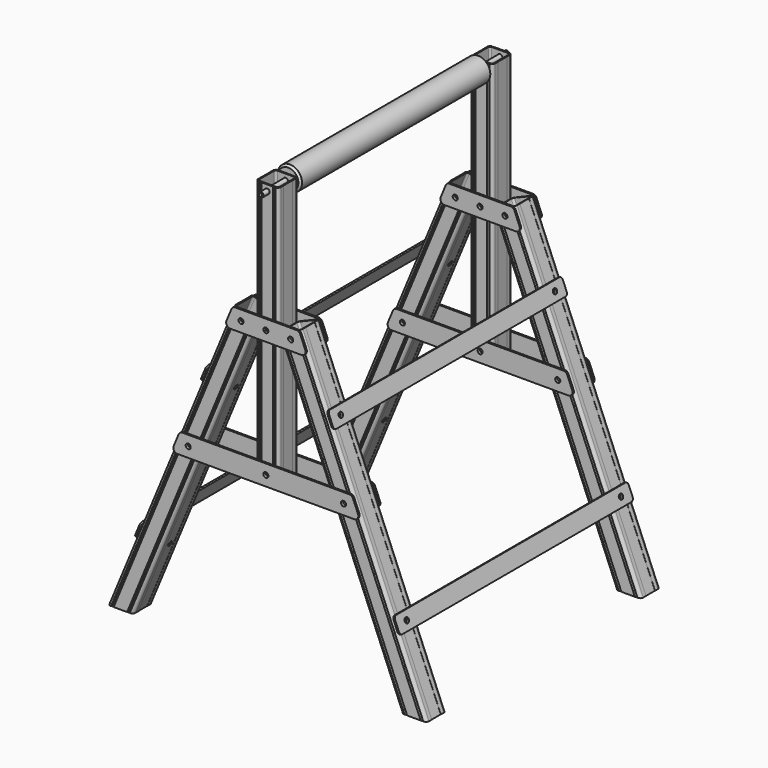
from build123d import *

# Parameters (mm, degrees)
F0_R      = 6.25
F1_DEPTH  = 60
F2_R      = 7.5
F4_REACH  = 887.042655099
F5_R      = 6.25
F6_DEPTH  = 57.7
F7_W      = 55.7
F7_H      = 653.8274706661
F7_R      = 6.25
F8_DEPTH  = 60
F9_R      = 7.5
F11_DEPTH = 653.8274706661
F14_R     = 6.25
F15_DEPTH = 4
F16_R     = 10
F16_2_R   = 10
F21_R     = 5.9
F22_DEPTH = 380
F23_R     = 30
F23_R_2   = 6.25
F24_DEPTH = 295
F25_SIZE  = 2
F26_SIZE  = 5
F28_W     = 720
F28_H     = 40
F28_R     = 6.25
F29_DEPTH = 4
F30_R     = 7.5
F30_2_R   = 7.5


# Not quite as in the source:
# - a feature names something its author has since deleted; it is built from what else it names


with BuildPart() as f1:
    # F0 (on Front) → F1 (new body)
    with BuildSketch(Plane.XZ):
        Polygon((-62.4540299569, 0), (0, 0), (-310.7389470805, 750.1901803992), (-364.0467961064, 728.1093463517), align=None)
        with Locations((-201.5402531038, 411.1725293339)):
            Circle(F0_R, mode=Mode.SUBTRACT)
        with Locations((-331.6526201079, 725.2915703878)):
            Circle(F0_R, mode=Mode.SUBTRACT)
    extrude(amount=F1_DEPTH)

    # F2
    f2_edges = [f1.edges().sort_by_distance(p)[0] for p in [
        (-155.369474, -60, 375.09509),
        (-213.250413, -60, 364.054673),
        (-155.369474, 0, 375.09509),
        (-213.250413, 0, 364.054673),
    ]]
    fillet(f2_edges, radius=F2_R)

    f4_end = f1.faces().sort_by_distance((-31.2270149784, -30, 0))[0]
    # F3 (on face) → F4 (cut, up to a face of the model that its end follows)
    with BuildSketch(Plane(origin=(-310.7389470805, 0, 750.1901803992), x_dir=(0.9238795325, 0, 0.3826834324), z_dir=(-0.3826834324, 0, 0.9238795325))):
        with BuildLine():
            Line((-54.8, -30), (-54.8, -52.5))
            ThreePointArc((-54.8, -52.5), (-53.4526911935, -55.7526911935), (-50.2, -57.1))
            Line((-50.2, -57.1), (-28.85, -57.1))
            Line((-28.85, -57.1), (-7.5, -57.1))
            ThreePointArc((-7.5, -57.1), (-4.2473088065, -55.7526911935), (-2.9, -52.5))
            Line((-2.9, -52.5), (-2.9, -30))
            Line((-2.9, -30), (-2.9, -7.5))
            ThreePointArc((-2.9, -7.5), (-4.2473088065, -4.2473088065), (-7.5, -2.9))
            Line((-7.5, -2.9), (-28.85, -2.9))
            Line((-28.85, -2.9), (-50.2, -2.9))
            ThreePointArc((-50.2, -2.9), (-53.4526911935, -4.2473088065), (-54.8, -7.5))
            Line((-54.8, -7.5), (-54.8, -30))
        make_face()
        Polygon((-44.2, 0), (-46.2, 0), (-45.2, -1), align=None)
        Polygon((-46.2, 0), (-48.2, 0), (-47.2, -1), align=None)
        Polygon((-48.2, 0), (-50.2, 0), (-49.2, -1), align=None)
        Polygon((-57.7, -16), (-57.7, -44), (-57.4, -44), (-57.4, -30), (-57.4, -16), align=None)
        Polygon((-49.2, -59), (-50.2, -60), (-48.2, -60), align=None)
        Polygon((-47.2, -59), (-48.2, -60), (-46.2, -60), align=None)
        Polygon((-45.2, -59), (-46.2, -60), (-44.2, -60), align=None)
        Polygon((-8.5, -59), (-9.5, -60), (-7.5, -60), align=None)
        Polygon((-10.5, -59), (-11.5, -60), (-9.5, -60), align=None)
        Polygon((-12.5, -59), (-13.5, -60), (-11.5, -60), align=None)
        Polygon((-0.3, -44), (0, -44), (0, -16), (-0.3, -16), (-0.3, -30), align=None)
        Polygon((-7.5, 0), (-9.5, 0), (-8.5, -1), align=None)
        Polygon((-9.5, 0), (-11.5, 0), (-10.5, -1), align=None)
        Polygon((-11.5, 0), (-13.5, 0), (-12.5, -1), align=None)
    f4_long = extrude(amount=-F4_REACH, mode=Mode.PRIVATE)
    add(split(f4_long, bisect_by=f4_end, keep=Keep.BOTTOM, mode=Mode.PRIVATE), mode=Mode.SUBTRACT)

    # F5 (on face) → F6 (cut, through all)
    with BuildSketch(Plane(origin=(0, 0, 0), x_dir=(0, 1, 0), z_dir=(0.9238795325, 0, 0.3826834324))):
        with Locations((-30, 200)):
            Circle(F5_R)
        with Locations((-30, 625)):
            Circle(F5_R)
    extrude(amount=-F6_DEPTH, mode=Mode.SUBTRACT)


with BuildPart() as f8:
    # F7 (on face) → F8 (new body)
    with BuildSketch(Plane.XZ.offset(60)):
        with Locations((-392.8967961064, 713.086264667)):
            Rectangle(F7_W, F7_H)
        with Locations((-392.8967961064, 411.1725293339)):
            Circle(F7_R, mode=Mode.SUBTRACT)
        with Locations((-392.8967961064, 725.2915703878)):
            Circle(F7_R, mode=Mode.SUBTRACT)
        with Locations((-392.8967961064, 1025)):
            Circle(F7_R, mode=Mode.SUBTRACT)
    extrude(amount=-F8_DEPTH)

    # F9
    f9_edges = [f8.edges().sort_by_distance(p)[0] for p in [
        (-420.746796, -60, 713.086265),
        (-365.046796, -60, 713.086265),
        (-365.046796, 0, 713.086265),
        (-420.746796, 0, 713.086265),
    ]]
    fillet(f9_edges, radius=F9_R)

    # F10 (on face) → F11 (cut, through all)
    with BuildSketch(Plane.XY.offset(1040)):
        Polygon((-412.2467961064, -59), (-413.2467961064, -60), (-411.2467961064, -60), align=None)
        Polygon((-410.2467961064, -59), (-411.2467961064, -60), (-409.2467961064, -60), align=None)
        Polygon((-408.2467961064, -59), (-409.2467961064, -60), (-407.2467961064, -60), align=None)
        Polygon((-377.5467961064, -59), (-378.5467961064, -60), (-376.5467961064, -60), align=None)
        Polygon((-375.5467961064, -59), (-376.5467961064, -60), (-374.5467961064, -60), align=None)
        Polygon((-373.5467961064, -59), (-374.5467961064, -60), (-372.5467961064, -60), align=None)
        Polygon((-420.7467961064, -16), (-420.7467961064, -44), (-420.4467961064, -44), (-420.4467961064, -30), (-420.4467961064, -16), align=None)
        Polygon((-365.3467961064, -44), (-365.0467961064, -44), (-365.0467961064, -16), (-365.3467961064, -16), (-365.3467961064, -30), align=None)
        Polygon((-376.5467961064, 0), (-378.5467961064, 0), (-377.5467961064, -1), align=None)
        Polygon((-374.5467961064, 0), (-376.5467961064, 0), (-375.5467961064, -1), align=None)
        Polygon((-372.5467961064, 0), (-374.5467961064, 0), (-373.5467961064, -1), align=None)
        Polygon((-411.2467961064, 0), (-413.2467961064, 0), (-412.2467961064, -1), align=None)
        Polygon((-409.2467961064, 0), (-411.2467961064, 0), (-410.2467961064, -1), align=None)
        Polygon((-407.2467961064, 0), (-409.2467961064, 0), (-408.2467961064, -1), align=None)
        with BuildLine():
            Line((-417.8467961064, -30), (-417.8467961064, -52.5))
            ThreePointArc((-417.8467961064, -52.5), (-416.4994872998, -55.7526911935), (-413.2467961064, -57.1))
            Line((-413.2467961064, -57.1), (-392.8967961064, -57.1))
            Line((-392.8967961064, -57.1), (-372.5467961064, -57.1))
            ThreePointArc((-372.5467961064, -57.1), (-369.2941049129, -55.7526911935), (-367.9467961064, -52.5))
            Line((-367.9467961064, -52.5), (-367.9467961064, -30))
            Line((-367.9467961064, -30), (-367.9467961064, -7.5))
            ThreePointArc((-367.9467961064, -7.5), (-369.2941049129, -4.2473088065), (-372.5467961064, -2.9))
            Line((-372.5467961064, -2.9), (-392.8967961064, -2.9))
            Line((-392.8967961064, -2.9), (-413.2467961064, -2.9))
            ThreePointArc((-413.2467961064, -2.9), (-416.4994872998, -4.2473088065), (-417.8467961064, -7.5))
            Line((-417.8467961064, -7.5), (-417.8467961064, -30))
        make_face()
    extrude(amount=-F11_DEPTH, mode=Mode.SUBTRACT)


with BuildPart() as f13_1:
    # F13: instance of F1
    add(f1.part.mirror(Plane(origin=(-392.8967961064, -30, 713.086264667), x_dir=(0, 1, 0), z_dir=(1, 0, 0))))


with BuildPart() as f15:
    # F14 (on face) → F15 (new body)
    with BuildSketch(Plane.XZ.offset(60)):
        Polygon((-180.6685771847, 436.1725293339), (-605.125015028, 436.1725293339), (-625.8356931467, 386.1725293339), (-159.957899066, 386.1725293339), align=None)
        with Locations((-584.2533391089, 411.1725293339)):
            Circle(F14_R, mode=Mode.SUBTRACT)
        with Locations((-392.8967961064, 411.1725293339)):
            Circle(F14_R, mode=Mode.SUBTRACT)
        with Locations((-201.5402531038, 411.1725293339)):
            Circle(F14_R, mode=Mode.SUBTRACT)
    extrude(amount=F15_DEPTH)

    # F16
    f16_edges = [f15.edges().sort_by_distance(p)[0] for p in [
        (-625.835693, -62, 386.172529),
        (-605.125015, -62, 436.172529),
        (-180.668577, -62, 436.172529),
        (-159.957899, -62, 386.172529),
    ]]
    fillet(f16_edges, radius=F16_R)


with BuildPart() as f15b:
    # F14 (on face) → F15, piece 2 (new body)
    with BuildSketch(Plane.XZ.offset(60)):
        Polygon((-310.7389470805, 750.1901803992), (-475.0546451323, 750.1901803992), (-495.7653232509, 700.1901803992), (-290.0282689618, 700.1901803992), align=None)
        with Locations((-454.1409721048, 725.2915703878)):
            Circle(F14_R, mode=Mode.SUBTRACT)
        with Locations((-392.8967961064, 725.1901803992)):
            Circle(F14_R, mode=Mode.SUBTRACT)
        with Locations((-331.6526201079, 725.2915703878)):
            Circle(F14_R, mode=Mode.SUBTRACT)
    extrude(amount=F15_DEPTH)

    # F16#2
    f16_2_edges = [f15b.edges().sort_by_distance(p)[0] for p in [
        (-475.054645, -62, 750.19018),
        (-495.765323, -62, 700.19018),
        (-310.738947, -62, 750.19018),
        (-290.028269, -62, 700.19018),
    ]]
    fillet(f16_2_edges, radius=F16_2_R)


with BuildPart() as f18_1:
    # F18: instance of F15
    add(f15.part.mirror(Plane(origin=(-392.8967961064, -30, 712.9824259225), x_dir=(1, 0, 0), z_dir=(0, -1, 0))))


with BuildPart() as f18_2:
    # F18: instance of F15b
    add(f15b.part.mirror(Plane(origin=(-392.8967961064, -30, 712.9824259225), x_dir=(1, 0, 0), z_dir=(0, -1, 0))))


with BuildPart() as f20_1:
    # F20: instance of F1
    add(f1.part.mirror(Plane(origin=(-392.8967961064, -360, 712.9381401651), x_dir=(1, 0, 0), z_dir=(0, -1, 0))))


with BuildPart() as f20_2:
    # F20: instance of F18_2
    add(f18_2.part.mirror(Plane(origin=(-392.8967961064, -360, 712.9381401651), x_dir=(1, 0, 0), z_dir=(0, -1, 0))))


with BuildPart() as f20_3:
    # F20: instance of F8
    add(f8.part.mirror(Plane(origin=(-392.8967961064, -360, 712.9381401651), x_dir=(1, 0, 0), z_dir=(0, -1, 0))))


with BuildPart() as f20_4:
    # F20: instance of F13_1
    add(f13_1.part.mirror(Plane(origin=(-392.8967961064, -360, 712.9381401651), x_dir=(1, 0, 0), z_dir=(0, -1, 0))))


with BuildPart() as f20_5:
    # F20: instance of F15
    add(f15.part.mirror(Plane(origin=(-392.8967961064, -360, 712.9381401651), x_dir=(1, 0, 0), z_dir=(0, -1, 0))))


with BuildPart() as f20_6:
    # F20: instance of F15b
    add(f15b.part.mirror(Plane(origin=(-392.8967961064, -360, 712.9381401651), x_dir=(1, 0, 0), z_dir=(0, -1, 0))))


with BuildPart() as f20_7:
    # F20: instance of F18_1
    add(f18_1.part.mirror(Plane(origin=(-392.8967961064, -360, 712.9381401651), x_dir=(1, 0, 0), z_dir=(0, -1, 0))))


with BuildPart() as f22:
    # F21 (on offset) → F22 (new body, symmetric)
    with BuildSketch(Plane.XZ.offset(360)):
        with Locations((-392.8967961064, 1025)):
            Circle(F21_R)
    extrude(amount=F22_DEPTH, both=True)

    # F25
    f25_edges = [f22.edges().sort_by_distance(p)[0] for p in [
        (-398.796796, 20, 1025),
        (-398.796796, -740, 1025),
    ]]
    chamfer(f25_edges, length=F25_SIZE)


with BuildPart() as f24:
    # F23 (on offset) → F24 (new body, symmetric)
    with BuildSketch(Plane.XZ.offset(360)):
        with Locations((-392.8967961064, 1025)):
            Circle(F23_R)
        with Locations((-392.8967961064, 1025)):
            Circle(F23_R_2, mode=Mode.SUBTRACT)
    extrude(amount=F24_DEPTH, both=True)

    # F26
    f26_edges = [f24.edges().sort_by_distance(p)[0] for p in [
        (-422.896796, -655, 1025),
        (-422.896796, -65, 1025),
    ]]
    chamfer(f26_edges, length=F26_SIZE)


with BuildPart() as f29:
    # F28 (on face) → F29 (new body)
    with BuildSketch(Plane(origin=(0, 0, 0), x_dir=(0, 1, 0), z_dir=(0.9238795325, 0, 0.3826834324))):
        with Locations((-360, 200)):
            Rectangle(F28_W, F28_H)
        with Locations((-690, 200)):
            Circle(F28_R, mode=Mode.SUBTRACT)
        with Locations((-30, 200)):
            Circle(F28_R, mode=Mode.SUBTRACT)
    extrude(amount=F29_DEPTH)

    # F30
    f30_edges = [f29.edges().sort_by_distance(p)[0] for p in [
        (-82.342596, 0, 204.018864),
        (-67.035259, 0, 167.063683),
        (-82.342596, -720, 204.018864),
        (-67.035259, -720, 167.063683),
    ]]
    fillet(f30_edges, radius=F30_R)


with BuildPart() as f29b:
    # F28 (on face) → F29, piece 2 (new body)
    with BuildSketch(Plane(origin=(0, 0, 0), x_dir=(0, 1, 0), z_dir=(0.9238795325, 0, 0.3826834324))):
        with Locations((-360, 625)):
            Rectangle(F28_W, F28_H)
        with Locations((-690, 625)):
            Circle(F28_R, mode=Mode.SUBTRACT)
        with Locations((-30, 625)):
            Circle(F28_R, mode=Mode.SUBTRACT)
    extrude(amount=F29_DEPTH)

    # F30#2
    f30_2_edges = [f29b.edges().sort_by_distance(p)[0] for p in [
        (-244.983055, -720, 596.667665),
        (-229.675718, -720, 559.712484),
        (-244.983055, 0, 596.667665),
        (-229.675718, 0, 559.712484),
    ]]
    fillet(f30_2_edges, radius=F30_2_R)


with BuildPart() as f31_1:
    # F31: instance of F29
    add(f29.part.mirror(Plane(origin=(-392.8967961064, -30, 713.086264667), x_dir=(0, 1, 0), z_dir=(1, 0, 0))))


with BuildPart() as f31_2:
    # F31: instance of F29b
    add(f29b.part.mirror(Plane(origin=(-392.8967961064, -30, 713.086264667), x_dir=(0, 1, 0), z_dir=(1, 0, 0))))


solid = Compound([f1.part, f8.part, f13_1.part, f15.part, f15b.part, f18_1.part, f18_2.part, f20_1.part, f20_2.part, f20_3.part, f20_4.part, f20_5.part, f20_6.part, f20_7.part, f22.part, f24.part, f29.part, f29b.part, f31_1.part, f31_2.part])
